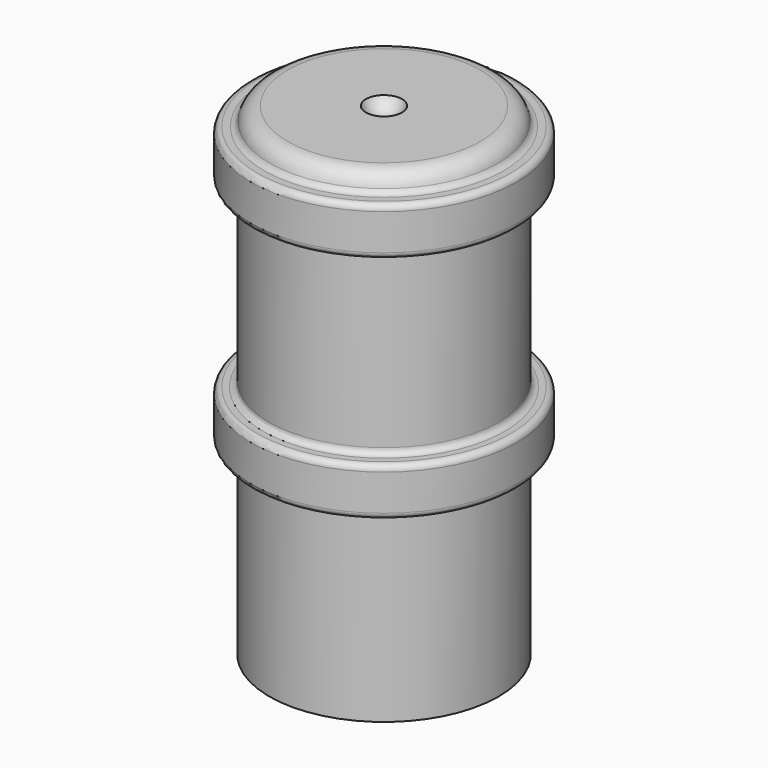
from build123d import *

# Parameters (mm, degrees)
F2_R = 0.5
F3_R = 0.5


with BuildPart() as f1:
    # F0 (on Front) → F1 (revolve)
    with BuildSketch(Plane.XZ):
        with BuildLine():
            Line((-9.5, -16.7268847123), (-8.65, -16.7268847123))
            Line((-8.65, -16.7268847123), (-8.3372622873, 9.334591348))
            Line((-8.3372622873, 9.334591348), (-8.3219749356, 10.6085373182))
            Line((-8.3219749356, 10.6085373182), (-8.2, 20.7731152877))
            Line((-8.2, 20.7731152877), (0, 20.7731152877))
            Line((0, 20.7731152877), (0, 22.2731152877))
            ThreePointArc((0, 22.2731152877), (-0.9013878189, 22.5460335594), (-1.5, 23.2731152877))
            Line((-1.5, 23.2731152877), (-8, 23.2731152877))
            ThreePointArc((-8, 23.2731152877), (-9.0606601718, 22.8337754595), (-9.5, 21.7731152877))
            Line((-9.5, 21.7731152877), (-11, 21.7731152877))
            Line((-11, 21.7731152877), (-11, 17.7731152877))
            Line((-11, 17.7731152877), (-9.5, 17.7731152877))
            Line((-9.5, 17.7731152877), (-9.5, 2.7731152877))
            Line((-9.5, 2.7731152877), (-11, 2.7731152877))
            Line((-11, 2.7731152877), (-11, -1.2268847123))
            Line((-11, -1.2268847123), (-9.5, -1.2268847123))
            Line((-9.5, -1.2268847123), (-9.5, -16.7268847123))
        make_face()
    revolve(axis=Axis((0, 0, 4.3270599525), (0, 0, -1)))

    # F2
    f2_edges = [f1.edges().sort_by_distance(p)[0] for p in [
        (11, 0, 21.773115),
        (11, 0, 17.773115),
        (11, 0, 2.773115),
        (11, 0, -1.226885),
    ]]
    fillet(f2_edges, radius=F2_R)

    # F3
    f3_edges = [f1.edges().sort_by_distance(p)[0] for p in [
        (9.5, 0, 17.773115),
        (9.5, 0, 2.773115),
        (9.5, 0, 21.773115),
        (9.5, 0, -1.226885),
    ]]
    fillet(f3_edges, radius=F3_R)


with BuildPart() as f1b:
    # F0 (on Front) → F1, piece 2 (revolve)
    with BuildSketch(Plane.XZ):
        with BuildLine():
            ThreePointArc((-7.8088648302, 9.9731152877), (-7.9531581803, 10.381478832), (-8.3219749356, 10.6085373182))
            Line((-8.3219749356, 10.6085373182), (-8.3219749356, 9.9731152877))
            Line((-8.3219749356, 9.9731152877), (-7.8088648302, 9.9731152877))
        make_face()
    revolve(axis=Axis((0, 0, 4.3270599525), (0, 0, -1)))


with BuildPart() as f4:
    # F0 (on Front) → F4 (revolve)
    with BuildSketch(Plane.XZ):
        with BuildLine():
            Line((9.1536324471, 10.6085373182), (-8.3219749356, 10.6085373182))
            ThreePointArc((-8.3219749356, 10.6085373182), (-7.9531581803, 10.381478832), (-7.8088648302, 9.9731152877))
            Line((-7.8088648302, 9.9731152877), (9.1536324471, 9.9731152877))
            Line((9.1536324471, 9.9731152877), (9.1536324471, 10.6085373182))
        make_face()
    revolve(axis=Axis((0.4158287557, 0, 9.9731152877), (1, 0, 0)))


solid = Compound([f1.part, f1b.part, f4.part])
